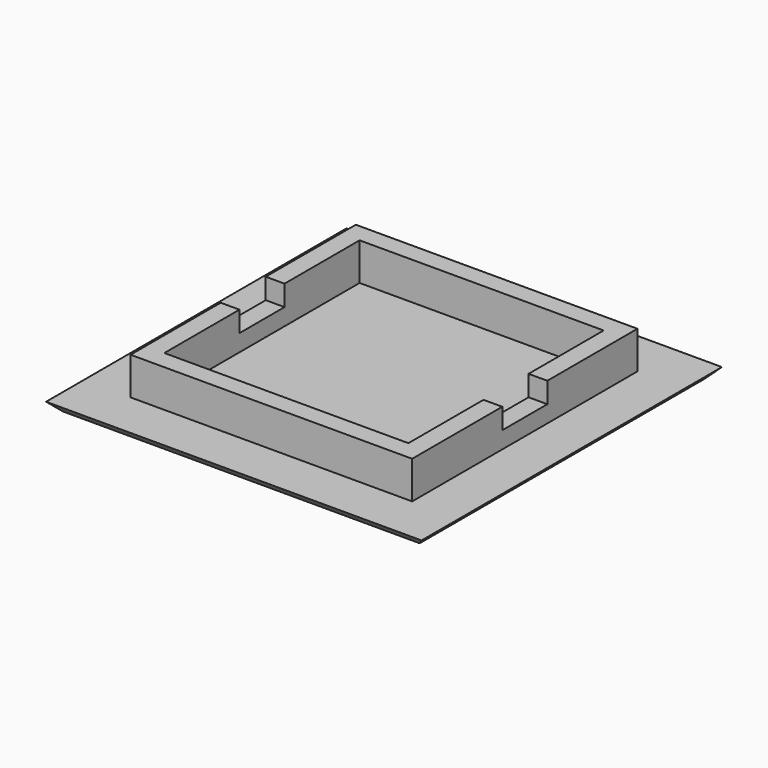
from build123d import *

# Parameters (mm, degrees)
F0_W     = 30
F0_H     = 30
F0_W_2   = 26
F0_H_2   = 26
F1_DEPTH = 5
F0_W_3   = 39.9999991059
F0_H_3   = 39.9999991059
F2_DEPTH = 1
F3_W     = 2
F3_H     = 6
F3_W_2   = 26
F4_DEPTH = 2.2
F6_SIZE  = 0.99999


# Not quite as in the source:
# - a fillet or chamfer is up to 0.001 mm smaller than in the source, because OpenCascade refuses the exact size
# - a feature of the source that left no trace in its solid (it failed there, or was rolled back) is left out


with BuildPart() as f1:
    # F0 (on Top) → F1 (new body)
    with BuildSketch(Plane.XY):
        Rectangle(F0_W, F0_H)
        Rectangle(F0_W_2, F0_H_2, mode=Mode.SUBTRACT)
    extrude(amount=F1_DEPTH)

    # F0 (on Top) → F2 (join)
    with BuildSketch(Plane.XY):
        Rectangle(F0_W_3, F0_H_3)
        Rectangle(F0_W, F0_H, mode=Mode.SUBTRACT)
        Rectangle(F0_W_2, F0_H_2)
    extrude(amount=F2_DEPTH)

    # F3 (on face) → F4 (cut)
    with BuildSketch(Plane.XY.offset(5)):
        with Locations((-14, 0)):
            Rectangle(F3_W, F3_H)
        Rectangle(F3_W_2, F3_H)
        with Locations((14, 0)):
            Rectangle(F3_W, F3_H)
    extrude(amount=-F4_DEPTH, mode=Mode.SUBTRACT)

    # F6 (size 1 in the source; OpenCascade refuses exactly that, so slightly less here)
    f6_edges = [f1.edges().sort_by_distance(p)[0] for p in [
        (-20, 0, 0),
        (0, -20, 0),
        (20, 0, 0),
        (0, 20, 0),
    ]]
    chamfer(f6_edges, length=F6_SIZE)


solid = f1.part
